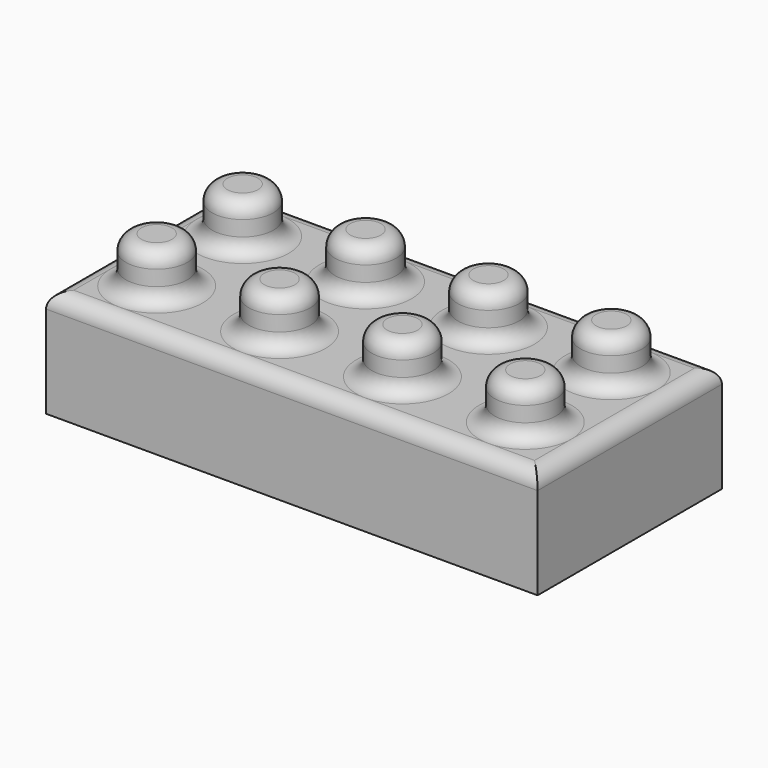
from build123d import *

# Parameters (mm, degrees)
F0_W     = 32
F0_H     = 15
F1_DEPTH = 7
F2_R     = 2
F3_DEPTH = 3
F4_R     = 0.99999


# Not quite as in the source:
# - a fillet or chamfer is up to 0.001 mm smaller than in the source, because OpenCascade refuses the exact size


with BuildPart() as f1:
    # F0 (on Top) → F1 (new body)
    with BuildSketch(Plane.XY):
        Rectangle(F0_W, F0_H)
    extrude(amount=F1_DEPTH)

    # F2 (on face) → F3 (join)
    with BuildSketch(Plane.XY.offset(7)):
        with Locations((-12, 3.5)):
            Circle(F2_R)
        with Locations((-12, -3.5)):
            Circle(F2_R)
        with Locations((-4, 3.5)):
            Circle(F2_R)
        with Locations((-4, -3.5)):
            Circle(F2_R)
        with Locations((4, -3.5)):
            Circle(F2_R)
        with Locations((4, 3.5)):
            Circle(F2_R)
        with Locations((12, 3.5)):
            Circle(F2_R)
        with Locations((12, -3.5)):
            Circle(F2_R)
    extrude(amount=F3_DEPTH)

    # F4 (radius 1 in the source; OpenCascade refuses exactly that, so slightly less here)
    f4_edges = [f1.edges().sort_by_distance(p)[0] for p in [
        (0, 7.5, 7),
        (16, 0, 7),
        (-16, 0, 7),
        (0, -7.5, 7),
        (-14, -3.5, 7),
        (-6, -3.5, 7),
        (2, -3.5, 7),
        (10, -3.5, 7),
        (-14, 3.5, 7),
        (-6, 3.5, 7),
        (2, 3.5, 7),
        (10, 3.5, 7),
        (-14, -3.5, 10),
        (-14, 3.5, 10),
        (-6, 3.5, 10),
        (-6, -3.5, 10),
        (2, -3.5, 10),
        (2, 3.5, 10),
        (10, 3.5, 10),
        (10, -3.5, 10),
    ]]
    fillet(f4_edges, radius=F4_R)


solid = f1.part
